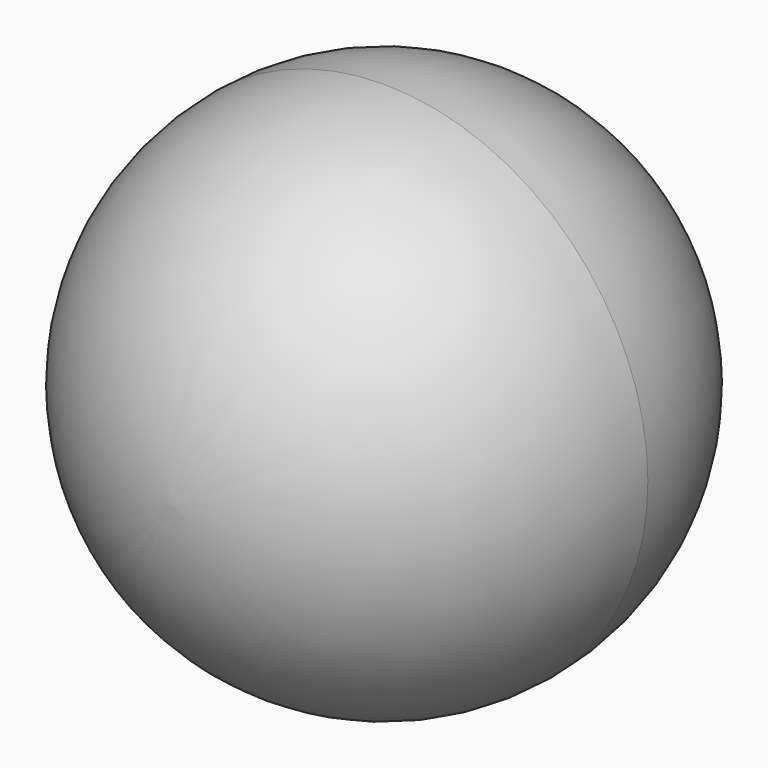
from build123d import *

# Parameters (mm, degrees)
F0_R     = 16.25
F1_DEPTH = 32.5
F2_R     = 16.24999


# Not quite as in the source:
# - a fillet or chamfer is up to 0.001 mm smaller than in the source, because OpenCascade refuses the exact size


with BuildPart() as f1:
    # F0 (on Front) → F1 (new body)
    with BuildSketch(Plane.XZ):
        Circle(F0_R)
    extrude(amount=F1_DEPTH)

    # F2 (radius 16.25 in the source; OpenCascade refuses exactly that, so slightly less here)
    f2_edges = [f1.edges().sort_by_distance(p)[0] for p in [
        (-16.25, -32.5, 0),
        (-16.25, 0, 0),
    ]]
    fillet(f2_edges, radius=F2_R)


solid = f1.part
